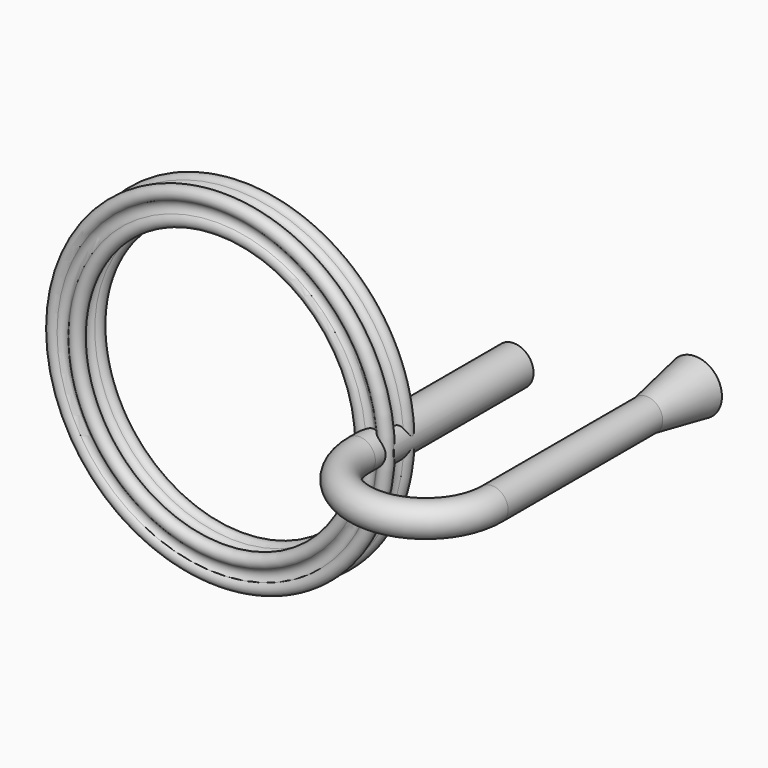
from build123d import *

# Parameters (mm, degrees)
F4_R      = 1.0577230165
F5_FACE_R = 1.0577230165
F6_DEPTH  = 4
F6_TAPER  = -10
F7_R      = 1.2981187366
F8_DEPTH  = 11.5


# Not quite as in the source:
# - a feature names something its author has since deleted; it is built from what else it names


with BuildPart() as f1:
    # F0 (on Top) → F1 (revolve)
    with BuildSketch(Plane.XY):
        with BuildLine():
            ThreePointArc((10.5592885973, 1.0362075193), (10.1858704224, 0.8373227652), (9.8124522476, 1.0362075193))
            ThreePointArc((9.8124522476, 1.0362075193), (9.1041893503, 1.0574581364), (9.2533454653, 0.3647530232))
            ThreePointArc((9.2533454653, 0.3647530232), (9.4996070634, -0.0364833953), (9.2533454653, -0.4377198139))
            ThreePointArc((9.2533454653, -0.4377198139), (9.1041893503, -1.1304249271), (9.8124522476, -1.1091743099))
            ThreePointArc((9.8124522476, -1.1091743099), (10.1858704224, -0.9102895558), (10.5592885973, -1.1091743099))
            ThreePointArc((10.5592885973, -1.1091743099), (11.2676306359, -1.1304690792), (11.1182975643, -0.4377198139))
            ThreePointArc((11.1182975643, -0.4377198139), (10.8720359662, -0.0364833953), (11.1182975643, 0.3647530232))
            ThreePointArc((11.1182975643, 0.3647530232), (11.2676306359, 1.0575022886), (10.5592885973, 1.0362075193))
        make_face()
    revolve(axis=Axis((0, 2.4106169393, 0), (0, 1, 0)))

    # F5: sweep along a path in F2
    with BuildLine(Plane.XY) as f5_path:
        Line((18.8743826002, 10.6943976134), (18.8743826002, -2.0534822252))
        ThreePointArc((18.8743826002, -2.0534822252), (14.5004992373, -6.427365588), (10.1266158745, -2.0534822252))
        Line((10.1266158745, -2.0534822252), (10.1266158745, -0.6472322857))
    # F4 (on line) → F5 (sweep)
    with BuildSketch(Plane(origin=(0, 10.6943976134, 0), x_dir=(-1, 0, 0), z_dir=(0, 1, 0))):
        with Locations((-18.8739430159, 0)):
            Circle(F4_R)
    sweep(path=f5_path.line)

    # F5_face (on face) → F6 (join)
    with BuildSketch(Plane(origin=(18.8739430159, 10.6943976134, 0), x_dir=(-1, 0, 0), z_dir=(0, 1, 0))):
        Circle(F5_FACE_R)
    extrude(amount=F6_DEPTH, taper=F6_TAPER)

    # F7 (on line) → F8 (join)
    with BuildSketch(Plane(origin=(0, 10.6943976134, 0), x_dir=(-1, 0, 0), z_dir=(0, 1, 0))):
        with Locations((-10.1158032194, 0)):
            Circle(F7_R)
    extrude(amount=-F8_DEPTH)


solid = f1.part
